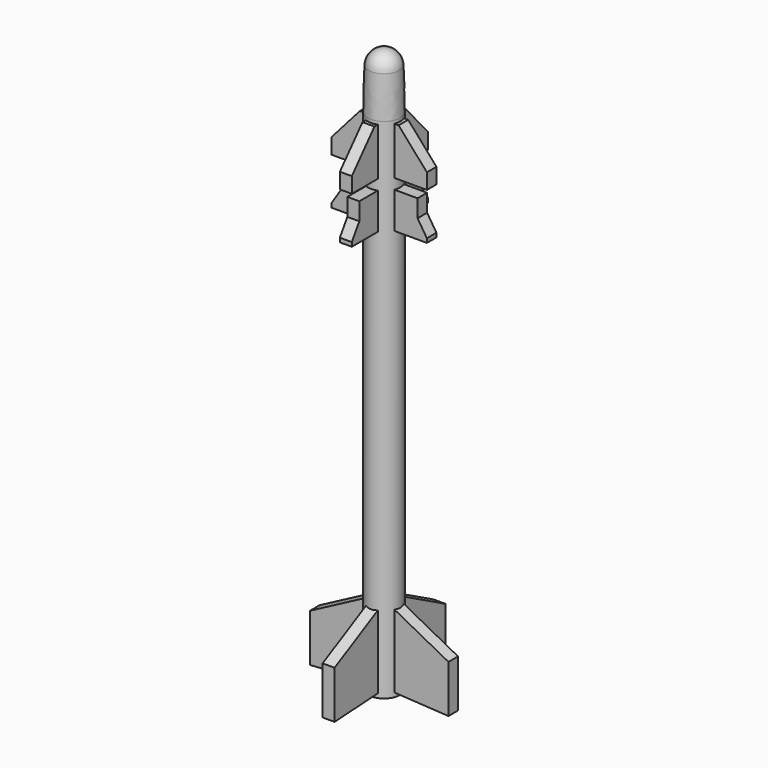
from build123d import *

# Parameters (mm, degrees)
F3_DEPTH = 0.2
F4_COUNT = 4


# Not quite as in the source:
# - a feature names something its author has since deleted; it is built from what else it names


with BuildPart() as f1:
    # F0 (on Front) → F1 (revolve)
    with BuildSketch(Plane.XZ):
        with BuildLine():
            Line((0, 18.8888888889), (0, 0))
            Line((0, 0), (0.5451388889, 0))
            Line((0.5451388889, 0), (0.5451388889, 17.0138888889))
            ThreePointArc((0.5451388889, 17.0138888889), (0.53654676, 17.7085458509), (0.5107756304, 18.4027777778))
            ThreePointArc((0.5107756304, 18.4027777778), (0.3525605469, 18.7479364578), (0, 18.8888888889))
        make_face()
    revolve(axis=Axis((0, 0, 9.4444444444), (0, 0, 1)))

    # F2 (on Front) → F3 (join, symmetric)
    with BuildSketch(Plane.XZ):
        Polygon((0, 16.9097222222), (0, 0.1708931289), (2.3194444444, 0.0347222222), (2.3194444444, 1.6319444444), (0.4, 2.6461323114), (0.4, 13.75), (1.5972222222, 13.75), (1.5972222222, 13.8888888889), (1.2847222222, 14.375), (1.2847222222, 14.9652777778), (0.4, 14.9652777778), (0.4, 15.3125), (1.5972222222, 15.3125), (1.5972222222, 15.8333333333), (0.6493055556, 16.9097222222), align=None)
    extrude(amount=F3_DEPTH, both=True)

    # F4: F1 ×4 about axis
    f4_axis = Axis((0, 0, 0), (0, 0, 1))


with BuildPart() as f1_1:
    add(f1.part)
    for i in range(1, F4_COUNT):
        add(f1.part.rotate(f4_axis, i * 360 / F4_COUNT))


solid = f1_1.part
